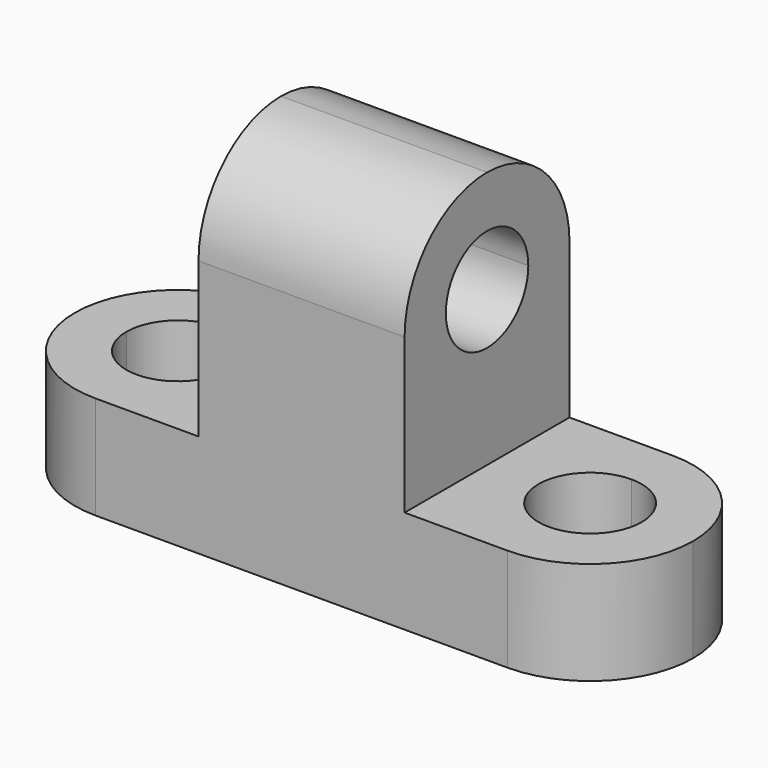
from build123d import *

# Parameters (mm, degrees)
F1_DEPTH = 25.4
F3_DEPTH = 12.7
F5_DEPTH = 25.4
F7_DEPTH = 25.4
F9_DEPTH = 12.7


with BuildPart() as f1:
    # F0 (on Front) → F1 (new body)
    with BuildSketch(Plane.XZ):
        Polygon((-37.9636640911, -15.4334478322), (-50.6636640911, -15.4334478322), (-50.6636640911, -28.1334478322), (0.1363359089, -28.1334478322), (0.1363359089, -15.4334478322), (-12.5636640911, -15.4334478322), (-12.5636640911, 3.6165521678), (-37.9636640911, 3.6165521678), align=None)
    extrude(amount=F1_DEPTH)

    # F2 (on face) → F3 (join)
    with BuildSketch(Plane.XY.offset(-15.4334478322)):
        with BuildLine():
            ThreePointArc((12.8363359089, -12.7), (9.11659203, -3.7197438789), (0.1363359089, 0))
            Line((0.1363359089, 0), (0.1363359089, -12.7))
            Line((0.1363359089, -12.7), (12.8363359089, -12.7))
        make_face()
        with BuildLine():
            Line((12.8363359089, -12.7), (0.1363359089, -12.7))
            Line((0.1363359089, -12.7), (0.1363359089, -25.4))
            ThreePointArc((0.1363359089, -25.4), (9.11659203, -21.6802561211), (12.8363359089, -12.7))
        make_face()
        with BuildLine():
            Line((-50.6636640911, -12.7), (-50.6636640911, 0))
            ThreePointArc((-50.6636640911, 0), (-59.6439202122, -3.7197438789), (-63.3636640911, -12.7))
            Line((-63.3636640911, -12.7), (-50.6636640911, -12.7))
        make_face()
        with BuildLine():
            Line((-50.6636640911, -25.4), (-50.6636640911, -12.7))
            Line((-50.6636640911, -12.7), (-63.3636640911, -12.7))
            ThreePointArc((-63.3636640911, -12.7), (-59.6439202122, -21.6802561211), (-50.6636640911, -25.4))
        make_face()
    extrude(amount=-F3_DEPTH)

    # F4 (on face) → F5 (join)
    with BuildSketch(Plane.YZ.offset(-12.5636640911)):
        with BuildLine():
            ThreePointArc((-12.7, 16.3165521678), (-21.6802561211, 12.5968082888), (-25.4, 3.6165521678))
            Line((-25.4, 3.6165521678), (-12.7, 3.6165521678))
            Line((-12.7, 3.6165521678), (-12.7, 16.3165521678))
        make_face()
        with BuildLine():
            Line((-12.7, 16.3165521678), (-12.7, 3.6165521678))
            Line((-12.7, 3.6165521678), (0, 3.6165521678))
            ThreePointArc((0, 3.6165521678), (-3.7197438789, 12.5968082888), (-12.7, 16.3165521678))
        make_face()
    extrude(amount=-F5_DEPTH)

    # F6 (on face) → F7 (cut)
    with BuildSketch(Plane.YZ.offset(-12.5636640911)):
        with BuildLine():
            ThreePointArc((-6.35, 3.6165521678), (-8.2098719395, 8.1066802283), (-12.7, 9.9665521678))
            ThreePointArc((-12.7, 9.9665521678), (-17.1901280605, 8.1066802283), (-19.05, 3.6165521678))
            ThreePointArc((-19.05, 3.6165521678), (-12.7, -2.7334478322), (-6.35, 3.6165521678))
        make_face()
    extrude(amount=-F7_DEPTH, mode=Mode.SUBTRACT)

    # F8 (on face) → F9 (cut)
    with BuildSketch(Plane.XY.offset(-15.4334478322)):
        with BuildLine():
            ThreePointArc((-44.3136640911, -12.7), (-46.1735360306, -8.2098719395), (-50.6636640911, -6.35))
            ThreePointArc((-50.6636640911, -6.35), (-55.1537921516, -8.2098719395), (-57.0136640911, -12.7))
            ThreePointArc((-57.0136640911, -12.7), (-55.1537921516, -17.1901280605), (-50.6636640911, -19.05))
            ThreePointArc((-50.6636640911, -19.05), (-46.1735360306, -17.1901280605), (-44.3136640911, -12.7))
        make_face()
        with BuildLine():
            ThreePointArc((0.1363359089, -19.05), (4.6264639694, -17.1901280605), (6.4863359089, -12.7))
            ThreePointArc((6.4863359089, -12.7), (4.6264639694, -8.2098719395), (0.1363359089, -6.35))
            ThreePointArc((0.1363359089, -6.35), (-6.2136640911, -12.7), (0.1363359089, -19.05))
        make_face()
    extrude(amount=-F9_DEPTH, mode=Mode.SUBTRACT)


solid = f1.part
